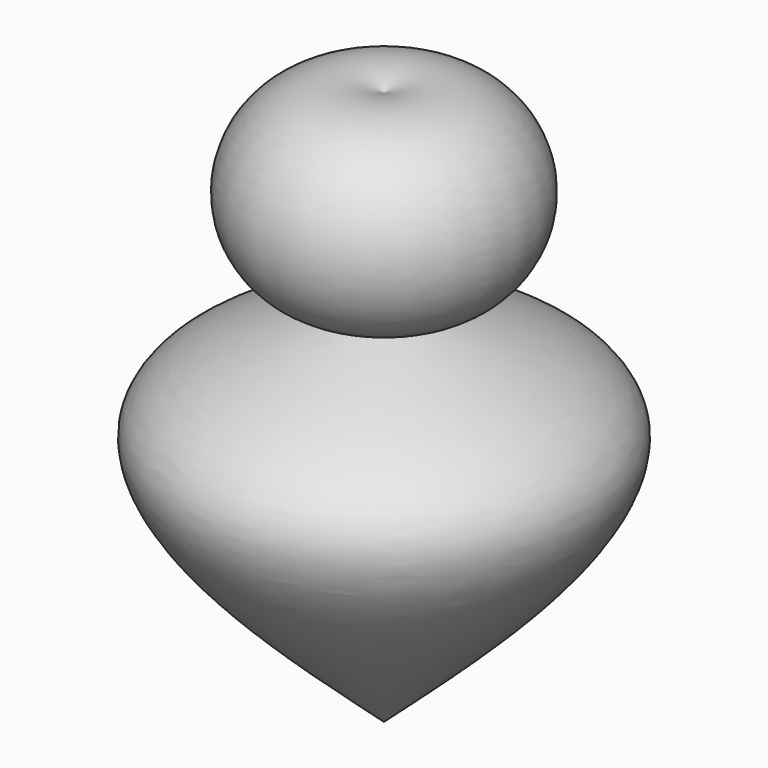
from build123d import *

# Parameters (mm, degrees)
F2_R     = 5.8477712981
F3_DEPTH = 25.4


with BuildPart() as f1:
    # F0 (on Right) → F1 (revolve)
    with BuildSketch(Plane.YZ):
        with BuildLine():
            add(Edge.make_bspline(
                [(-2.3902509112, 43.2604000923), (-12.9203770861, 39.8463630286), (-35.4506907368, 31.7121985459), (-12.7246468102, 11.3827549671), (0, 0)],
                knots=[0.0321341703, 0.0321341703, 0.0321341703, 0.0321341703, 0.4580776627, 1, 1, 1, 1], degree=3))
            Line((0, 0), (0, 44.0312027931))
            ThreePointArc((0, 44.0312027931), (-1.1732495857, 43.5779646048), (-2.3902509112, 43.2604000923))
        make_face()
    revolve(axis=Axis((0, 0, 32.1239307523), (0, 0, 1)))

    # F2 (on Top) → F3 (cut)
    with BuildSketch(Plane.XY):
        Circle(F2_R)
    extrude(amount=-F3_DEPTH, mode=Mode.SUBTRACT)


with BuildPart() as f1b:
    # F0 (on Right) → F1, piece 2 (revolve)
    with BuildSketch(Plane.YZ):
        with BuildLine():
            add(Edge.make_bspline(
                [(0, 44.0312027931), (-0.7979168183, 43.7745829015), (-1.5958336367, 43.5179630098), (-2.3902509112, 43.2604000923)],
                knots=[0, 0, 0, 0, 0.0321341703, 0.0321341703, 0.0321341703, 0.0321341703], degree=3))
            Line((0, 44.0312027931), (0, 64.2478615046))
            ThreePointArc((0, 64.2478615046), (-15.6049896856, 55.3952626356), (-2.3902509112, 43.2604000923))
        make_face()
    revolve(axis=Axis((0, 0, 32.1239307523), (0, 0, 1)))


solid = Compound([f1.part, f1b.part])
